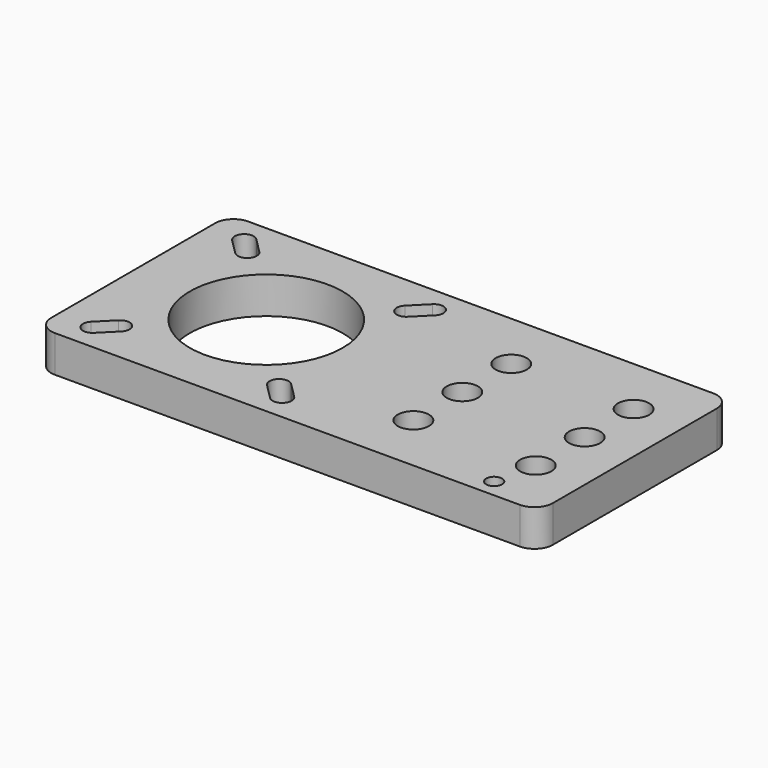
from build123d import *

# Parameters (mm, degrees)
F0_R     = 12.5
F0_R_2   = 2.55
F0_R_3   = 1.3
F1_DEPTH = 6


# Not quite as in the source:
# - ends of sketch curves that miss each other by under 0.0002 mm in the source are joined


with BuildPart() as f1:
    # F0 (on Top) → F1 (new body)
    with BuildSketch(Plane.XY):
        with BuildLine():
            Line((38, 19.75), (-38, 19.75))
            ThreePointArc((-38, 19.75), (-40.1213203436, 18.8713203436), (-41, 16.75))
            Line((-41, 16.75), (-41, -16.75))
            ThreePointArc((-41, -16.75), (-40.1213203436, -18.8713203436), (-38, -19.75))
            Line((-38, -19.75), (38, -19.75))
            ThreePointArc((38, -19.75), (40.1213203436, -18.8713203436), (41, -16.75))
            Line((41, -16.75), (41, 16.75))
            ThreePointArc((41, 16.75), (40.1213203436, 18.8713203436), (38, 19.75))
        make_face()
        with BuildLine():
            ThreePointArc((-34.1539839892, -16.5960150108), (-36.3460155108, -16.5960155108), (-36.3460150108, -14.4039839892))
            Line((-36.346015, -14.403984), (-33.846015, -11.903984))
            ThreePointArc((-33.8460150108, -11.9039839892), (-31.6539844892, -11.9039844892), (-31.6539839892, -14.0960150108))
            Line((-31.653984, -14.096015), (-34.153984, -16.596015))
        make_face(mode=Mode.SUBTRACT)
        with BuildLine():
            ThreePointArc((-3.1539844892, -14.4039844892), (-3.1539844892, -16.5960155108), (-5.3460155108, -16.5960155108))
            Line((-5.3460155108, -16.5960155108), (-7.846015, -14.096015))
            ThreePointArc((-7.846015, -14.096015), (-7.8460155108, -11.9039844892), (-5.6539844892, -11.9039844892))
            Line((-5.6539844892, -11.9039844892), (-3.1539844892, -14.4039844892))
        make_face(mode=Mode.SUBTRACT)
        with Locations((-19.25, 0)):
            Circle(F0_R, mode=Mode.SUBTRACT)
        with Locations((12.8, -10)):
            Circle(F0_R_2, mode=Mode.SUBTRACT)
        with Locations((31.4, -16.75)):
            Circle(F0_R_3, mode=Mode.SUBTRACT)
        with Locations((32.8, -10)):
            Circle(F0_R_2, mode=Mode.SUBTRACT)
        with Locations((12.8, 0)):
            Circle(F0_R_2, mode=Mode.SUBTRACT)
        with Locations((32.8, 0)):
            Circle(F0_R_2, mode=Mode.SUBTRACT)
        with BuildLine():
            ThreePointArc((-31.6539844892, 14.0960155108), (-31.6539844892, 11.9039844892), (-33.8460155108, 11.9039844892))
            Line((-33.8460155108, 11.9039844892), (-36.346015, 14.403985))
            ThreePointArc((-36.346015, 14.403985), (-36.3460155108, 16.5960155108), (-34.1539844892, 16.5960155108))
            Line((-34.1539844892, 16.5960155108), (-31.6539844892, 14.0960155108))
        make_face(mode=Mode.SUBTRACT)
        with BuildLine():
            ThreePointArc((-5.3460150108, 16.5960160108), (-3.1539844892, 16.5960155108), (-3.1539839892, 14.4039849892))
            Line((-3.153984, 14.403985), (-5.653984, 11.903985))
            ThreePointArc((-5.6539839892, 11.9039849892), (-7.8460155108, 11.9039844892), (-7.8460150108, 14.0960160108))
            Line((-7.846015, 14.096016), (-5.346015, 16.596016))
        make_face(mode=Mode.SUBTRACT)
        with Locations((12.8, 10)):
            Circle(F0_R_2, mode=Mode.SUBTRACT)
        with Locations((32.8, 10)):
            Circle(F0_R_2, mode=Mode.SUBTRACT)
    extrude(amount=F1_DEPTH)


solid = f1.part
